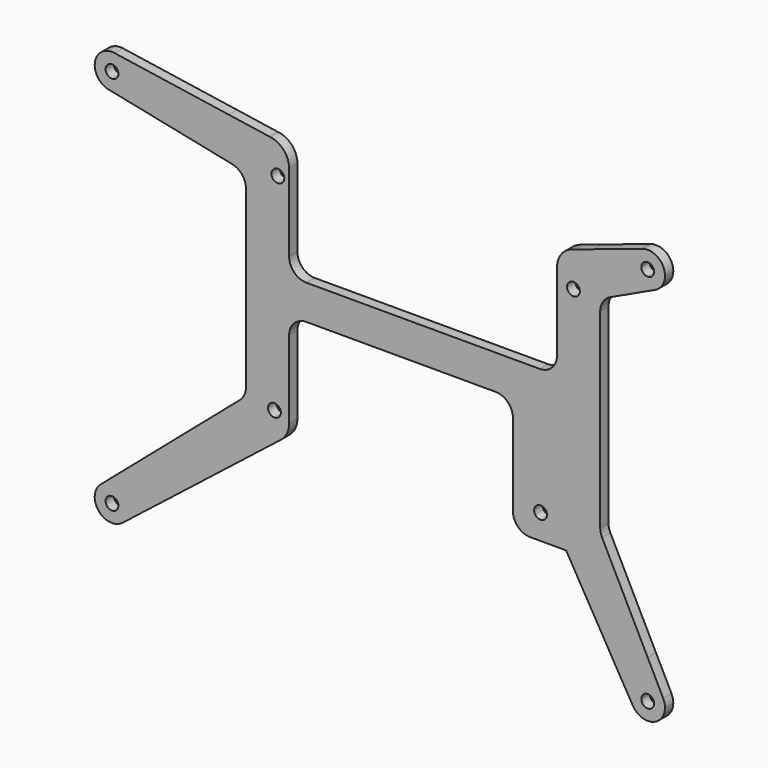
from build123d import *

# Parameters (mm, degrees)
F1_DEPTH = 3


# Not quite as in the source:
# - a feature names something its author has since deleted; it is built from what else it names


with BuildPart() as f1:
    # F0 (on Front) → F1 (new body)
    with BuildSketch(Plane.XZ):
        with BuildLine():
            Line((-37.214977254, 55.4332367199), (-65.9893809259, 55.4332367199))
            ThreePointArc((-65.9893809259, 55.4332367199), (-67.45384702, 51.8977028139), (-70.9893809259, 50.4332367199))
            Line((-70.9893809259, 50.4332367199), (-70.9893809259, 50.3281080825))
            Line((-70.9893809259, 50.3281080825), (-36.2299078147, 43.1628040761))
            ThreePointArc((-36.2299078147, 43.1628040761), (-33.3633413521, 41.4242986902), (-32.2393809259, 38.2657678257))
            Line((-32.2393809259, 38.2657678257), (-32.2393809259, -12.3991493743))
            ThreePointArc((-32.2393809259, -12.3991493743), (-32.6957967743, -14.4862150316), (-33.9817181489, -16.1922527517))
            Line((-33.9817181489, -16.1922527517), (-70.9893809259, -47.9758540661))
            Line((-70.9893809259, -47.9758540661), (-70.9893809259, -49.5667632801))
            ThreePointArc((-70.9893809259, -49.5667632801), (-67.45384702, -51.0312293742), (-65.9893809259, -54.5667632801))
            Line((-65.9893809259, -54.5667632801), (-62.9038139694, -54.5667632801))
            Line((-62.9038139694, -54.5667632801), (-22.1244695142, -22.4784798619))
            ThreePointArc((-22.1244695142, -22.4784798619), (-31.8953409933, -19.6117903415), (-25.9893809259, -11.3167632801))
            Line((-25.9893809259, -11.3167632801), (-25.9893809259, 41.1832367199))
            ThreePointArc((-25.9893809259, 41.1832367199), (-32.2393809259, 47.4332367199), (-25.9893809259, 53.6832367199))
            Line((-25.9893809259, 53.6832367199), (-25.5241895532, 53.6832367199))
            Line((-25.5241895532, 53.6832367199), (-37.214977254, 55.4332367199))
        make_face()
        with BuildLine():
            ThreePointArc((-70.2491754069, 60.3781427644), (-67.2011737249, 58.6965917729), (-65.9893809259, 55.4332367199))
            Line((-65.9893809259, 55.4332367199), (-37.214977254, 55.4332367199))
            Line((-37.214977254, 55.4332367199), (-70.2491754069, 60.3781427644))
        make_face()
        with BuildLine():
            ThreePointArc((-19.7393809259, 47.4332367199), (-21.2541219247, 51.5124305362), (-25.0641240271, 53.6143692756))
            ThreePointArc((-25.0641240271, 53.6143692756), (-25.5254727848, 53.6659960796), (-25.9893809259, 53.6832367199))
            ThreePointArc((-25.9893809259, 53.6832367199), (-32.2393809259, 47.4332367199), (-25.9893809259, 41.1832367199))
            ThreePointArc((-25.9893809259, 41.1832367199), (-21.5699635435, 43.0138193375), (-19.7393809259, 47.4332367199))
        make_face()
        with BuildLine():
            ThreePointArc((-21.1351809259, 44.4332367199), (-24.3004983196, 43.1221193262), (-22.9893809259, 46.2874367199))
            ThreePointArc((-22.9893809259, 46.2874367199), (-21.6782635322, 45.7443541135), (-21.1351809259, 44.4332367199))
        make_face(mode=Mode.SUBTRACT)
        with BuildLine():
            Line((-19.7393809259, 24.9332367629), (-19.7393809259, 47.4332367199))
            ThreePointArc((-19.7393809259, 47.4332367199), (-21.5699635435, 43.0138193375), (-25.9893809259, 41.1832367199))
            Line((-25.9893809259, 41.1832367199), (-25.9893809259, -11.3167632801))
            ThreePointArc((-25.9893809259, -11.3167632801), (-21.5699635435, -13.1473458977), (-19.7393809259, -17.5667632801))
            Line((-19.7393809259, -17.5667632801), (-19.7393809259, 4.9332367199))
            ThreePointArc((-19.7393809259, 4.9332367199), (-18.2749148318, 8.4687706258), (-14.7393809259, 9.9332367199))
            Line((-14.7393809259, 9.9332367199), (40.0127460063, 9.9332367199))
            ThreePointArc((40.0127460063, 9.9332367199), (43.5482799122, 8.4687706258), (45.0127460063, 4.9332367199))
            Line((45.0127460063, 4.9332367199), (45.0127460063, -17.5667632801))
            Line((45.0127460063, -17.5667632801), (51.449190997, -17.5667632801))
            ThreePointArc((51.449190997, -17.5667632801), (52.4896307348, -14.7872608805), (54.8648190741, -16.5667632801))
            ThreePointArc((54.8648190741, -16.5667632801), (54.7901214737, -17.0877516195), (54.5720471512, -17.5667632801))
            Line((54.5720471512, -17.5667632801), (57.7606190741, -17.5667632801))
            ThreePointArc((57.7606190741, -17.5667632801), (59.5912016917, -13.1473458977), (64.0106190741, -11.3167632801))
            Line((64.0106190741, -11.3167632801), (64.0106190741, 41.1832367199))
            ThreePointArc((64.0106190741, 41.1832367199), (59.5912016917, 43.0138193375), (57.7606190741, 47.4332367199))
            Line((57.7606190741, 47.4332367199), (57.7606190741, 24.9332367629))
            ThreePointArc((57.7606190741, 24.9332367629), (56.29615298, 21.3977028569), (52.7606190741, 19.9332367629))
            Line((52.7606190741, 19.9332367629), (-14.7393809259, 19.9332367629))
            ThreePointArc((-14.7393809259, 19.9332367629), (-18.2749148318, 21.3977028569), (-19.7393809259, 24.9332367629))
        make_face()
        with BuildLine():
            Line((-25.9893809259, -17.5667632801), (-25.9893809259, -11.3167632801))
            ThreePointArc((-25.9893809259, -11.3167632801), (-31.8953409933, -19.6117903415), (-22.1244695142, -22.4784798619))
            ThreePointArc((-22.1244695142, -22.4784798619), (-20.36718401, -20.2968551904), (-19.7393809259, -17.5667632801))
            Line((-19.7393809259, -17.5667632801), (-23.9893809259, -17.5667632801))
            Line((-23.9893809259, -17.5667632801), (-25.9893809259, -17.5667632801))
        make_face()
        with BuildLine():
            ThreePointArc((-19.7393809259, -17.5667632801), (-21.5699635435, -13.1473458977), (-25.9893809259, -11.3167632801))
            Line((-25.9893809259, -11.3167632801), (-25.9893809259, -17.5667632801))
            Line((-25.9893809259, -17.5667632801), (-23.9893809259, -17.5667632801))
            Line((-23.9893809259, -17.5667632801), (-19.7393809259, -17.5667632801))
        make_face()
        with BuildLine():
            ThreePointArc((-22.1351809259, -15.5667632801), (-22.6782635322, -16.8778806738), (-23.9893809259, -17.4209632801))
            ThreePointArc((-23.9893809259, -17.4209632801), (-25.3004983196, -14.2556458865), (-22.1351809259, -15.5667632801))
        make_face(mode=Mode.SUBTRACT)
        with BuildLine():
            Line((-62.9038139694, -54.5667632801), (-65.9893809259, -54.5667632801))
            ThreePointArc((-65.9893809259, -54.5667632801), (-66.4916233931, -56.7508368083), (-67.8974517965, -58.4961365456))
            Line((-67.8974517965, -58.4961365456), (-62.9038139694, -54.5667632801))
        make_face()
        with BuildLine():
            Line((-70.9893809259, -49.5667632801), (-70.9893809259, -47.9758540661))
            Line((-70.9893809259, -47.9758540661), (-74.2470437029, -50.7736599027))
            ThreePointArc((-74.2470437029, -50.7736599027), (-72.7264018114, -49.8781858367), (-70.9893809259, -49.5667632801))
        make_face()
        with BuildLine():
            Line((51.449190997, -17.5667632801), (45.0127460063, -17.5667632801))
            Line((45.0127460063, -17.5667632801), (45.0127460063, -18.8167632801))
            ThreePointArc((45.0127460063, -18.8167632801), (46.4772121003, -22.3522971861), (50.0127460063, -23.8167632801))
            Line((50.0127460063, -23.8167632801), (60.4091643842, -23.8167632801))
            Line((60.4091643842, -23.8167632801), (58.6032088142, -20.7008363936))
            ThreePointArc((58.6032088142, -20.7008363936), (57.974941228, -19.1894440675), (57.7606190741, -17.5667632801))
            Line((57.7606190741, -17.5667632801), (54.5720471512, -17.5667632801))
            ThreePointArc((54.5720471512, -17.5667632801), (53.0106190741, -18.4209632801), (51.449190997, -17.5667632801))
        make_face()
        with BuildLine():
            ThreePointArc((64.0106190741, 53.6832367199), (63.0073411856, 53.6021858588), (62.0300845889, 53.361135433))
            ThreePointArc((62.0300845889, 53.361135433), (58.9390887068, 51.0859178904), (57.7606190741, 47.4332367199))
            Line((57.7606190741, 47.4332367199), (64.0106190741, 47.4332367199))
            Line((64.0106190741, 47.4332367199), (70.2606190741, 47.4332367199))
            ThreePointArc((70.2606190741, 47.4332367199), (68.4300364565, 51.8526541023), (64.0106190741, 53.6832367199))
        make_face()
        with BuildLine():
            Line((82.4261914859, 60.1755556903), (68.2320500904, 55.4332367199))
            Line((68.2320500904, 55.4332367199), (79.0106190741, 55.4332367199))
            ThreePointArc((79.0106190741, 55.4332367199), (79.9533947803, 58.3553816563), (82.4261914859, 60.1755556903))
        make_face()
        with BuildLine():
            Line((79.0106190741, 55.4332367199), (68.2320500904, 55.4332367199))
            Line((68.2320500904, 55.4332367199), (62.9941595991, 53.6832367199))
            Line((62.9941595991, 53.6832367199), (64.0106190741, 53.6832367199))
            ThreePointArc((64.0106190741, 53.6832367199), (68.4300364565, 51.8526541023), (70.2606190741, 47.4332367199))
            Line((70.2606190741, 47.4332367199), (78.7288252988, 47.4332367199))
            Line((78.7288252988, 47.4332367199), (84.0106190741, 49.9105738121))
            Line((84.0106190741, 49.9105738121), (84.0106190741, 50.4332367199))
            ThreePointArc((84.0106190741, 50.4332367199), (80.4750851682, 51.8977028139), (79.0106190741, 55.4332367199))
        make_face()
        with BuildLine():
            Line((78.7288252988, 47.4332367199), (70.2606190741, 47.4332367199))
            ThreePointArc((70.2606190741, 47.4332367199), (68.4300364565, 43.0138193375), (64.0106190741, 41.1832367199))
            Line((64.0106190741, 41.1832367199), (64.0106190741, -11.3167632801))
            ThreePointArc((64.0106190741, -11.3167632801), (68.4300364565, -13.1473458977), (70.2606190741, -17.5667632801))
            ThreePointArc((70.2606190741, -17.5667632801), (68.4300364565, -21.9861806625), (64.0106190741, -23.8167632801))
            Line((64.0106190741, -23.8167632801), (60.4091643842, -23.8167632801))
            Line((60.4091643842, -23.8167632801), (78.2315125337, -54.5667632801))
            Line((78.2315125337, -54.5667632801), (79.0106190741, -54.5667632801))
            ThreePointArc((79.0106190741, -54.5667632801), (80.4750851682, -51.0312293742), (84.0106190741, -49.5667632801))
            Line((84.0106190741, -49.5667632801), (84.0106190741, -43.4349288765))
            Line((84.0106190741, -43.4349288765), (70.7933680849, -17.1438614305))
            ThreePointArc((70.7933680849, -17.1438614305), (70.3956290974, -16.0521179023), (70.2606190741, -14.898050085))
            Line((70.2606190741, -14.898050085), (70.2606190741, 40.2838696489))
            ThreePointArc((70.2606190741, 40.2838696489), (71.0406603386, 42.965650451), (73.1373983825, 44.810671378))
            Line((73.1373983825, 44.810671378), (78.7288252988, 47.4332367199))
        make_face()
        with BuildLine():
            Line((64.0106190741, 47.4332367199), (57.7606190741, 47.4332367199))
            ThreePointArc((57.7606190741, 47.4332367199), (59.5912016917, 43.0138193375), (64.0106190741, 41.1832367199))
            Line((64.0106190741, 41.1832367199), (64.0106190741, 42.3432561512))
            ThreePointArc((64.0106190741, 42.3432561512), (60.6564190741, 43.4332367199), (64.0106190741, 44.5232172885))
            Line((64.0106190741, 44.5232172885), (64.0106190741, 47.4332367199))
        make_face()
        with BuildLine():
            Line((64.0106190741, -17.5667632801), (64.0106190741, -11.3167632801))
            ThreePointArc((64.0106190741, -11.3167632801), (59.5912016917, -13.1473458977), (57.7606190741, -17.5667632801))
            Line((57.7606190741, -17.5667632801), (64.0106190741, -17.5667632801))
        make_face()
        with BuildLine():
            ThreePointArc((70.2606190741, -17.5667632801), (68.4300364565, -13.1473458977), (64.0106190741, -11.3167632801))
            Line((64.0106190741, -11.3167632801), (64.0106190741, -17.5667632801))
            Line((64.0106190741, -17.5667632801), (57.7606190741, -17.5667632801))
            ThreePointArc((57.7606190741, -17.5667632801), (57.974941228, -19.1894440675), (58.6032088142, -20.7008363936))
            ThreePointArc((58.6032088142, -20.7008363936), (60.8901589285, -22.9820406026), (64.0106190741, -23.8167632801))
            ThreePointArc((64.0106190741, -23.8167632801), (68.4300364565, -21.9861806625), (70.2606190741, -17.5667632801))
        make_face()
        with BuildLine():
            Line((58.6032088142, -20.7008363936), (60.4091643842, -23.8167632801))
            Line((60.4091643842, -23.8167632801), (64.0106190741, -23.8167632801))
            ThreePointArc((64.0106190741, -23.8167632801), (60.8901589285, -22.9820406026), (58.6032088142, -20.7008363936))
        make_face()
        with BuildLine():
            Line((88.4778700633, -52.3209519346), (84.0106190741, -43.4349288765))
            Line((84.0106190741, -43.4349288765), (84.0106190741, -49.5667632801))
            ThreePointArc((84.0106190741, -49.5667632801), (86.6346372974, -50.3106466976), (88.4778700633, -52.3209519346))
        make_face()
        with BuildLine():
            ThreePointArc((-70.9893809259, 53.5790367199), (-72.3004983196, 56.7443541135), (-69.1351809259, 55.4332367199))
            Line((-69.1351809259, 55.4332367199), (-65.9893809259, 55.4332367199))
            ThreePointArc((-65.9893809259, 55.4332367199), (-67.2011737249, 58.6965917729), (-70.2491754069, 60.3781427644))
            ThreePointArc((-70.2491754069, 60.3781427644), (-75.9121934648, 56.3084033935), (-71.9988540371, 50.5362004695))
            ThreePointArc((-71.9988540371, 50.5362004695), (-71.4967361998, 50.4590442602), (-70.9893809259, 50.4332367199))
            Line((-70.9893809259, 50.4332367199), (-70.9893809259, 53.5790367199))
        make_face()
        with BuildLine():
            Line((-65.9893809259, 55.4332367199), (-69.1351809259, 55.4332367199))
            ThreePointArc((-69.1351809259, 55.4332367199), (-69.6782635322, 54.1221193262), (-70.9893809259, 53.5790367199))
            Line((-70.9893809259, 53.5790367199), (-70.9893809259, 50.4332367199))
            ThreePointArc((-70.9893809259, 50.4332367199), (-67.45384702, 51.8977028139), (-65.9893809259, 55.4332367199))
        make_face()
        with BuildLine():
            ThreePointArc((82.4261914859, 60.1755556903), (79.9533947803, 58.3553816563), (79.0106190741, 55.4332367199))
            Line((79.0106190741, 55.4332367199), (82.1564190741, 55.4332367199))
            ThreePointArc((82.1564190741, 55.4332367199), (84.0106190741, 57.2874367199), (85.8648190741, 55.4332367199))
            ThreePointArc((85.8648190741, 55.4332367199), (85.3217364678, 54.1221193262), (84.0106190741, 53.5790367199))
            Line((84.0106190741, 53.5790367199), (84.0106190741, 50.4332367199))
            ThreePointArc((84.0106190741, 50.4332367199), (85.0982751214, 50.5529698908), (86.1338397657, 50.9064349908))
            ThreePointArc((86.1338397657, 50.9064349908), (88.2305778096, 52.7514559177), (89.0106190741, 55.4332367199))
            ThreePointArc((89.0106190741, 55.4332367199), (86.9327640105, 59.4904610137), (82.4261914859, 60.1755556903))
        make_face()
        with BuildLine():
            Line((82.1564190741, 55.4332367199), (79.0106190741, 55.4332367199))
            ThreePointArc((79.0106190741, 55.4332367199), (80.4750851682, 51.8977028139), (84.0106190741, 50.4332367199))
            Line((84.0106190741, 50.4332367199), (84.0106190741, 53.5790367199))
            ThreePointArc((84.0106190741, 53.5790367199), (82.6995016804, 54.1221193262), (82.1564190741, 55.4332367199))
        make_face()
        with BuildLine():
            ThreePointArc((-65.9893809259, -54.5667632801), (-67.45384702, -51.0312293742), (-70.9893809259, -49.5667632801))
            Line((-70.9893809259, -49.5667632801), (-70.9893809259, -52.7125632801))
            ThreePointArc((-70.9893809259, -52.7125632801), (-69.6782635322, -53.2556458865), (-69.1351809259, -54.5667632801))
            Line((-69.1351809259, -54.5667632801), (-65.9893809259, -54.5667632801))
        make_face()
        with BuildLine():
            Line((-70.9893809259, -52.7125632801), (-70.9893809259, -49.5667632801))
            ThreePointArc((-70.9893809259, -49.5667632801), (-72.7264018114, -49.8781858367), (-74.2470437029, -50.7736599027))
            ThreePointArc((-74.2470437029, -50.7736599027), (-74.8515083558, -57.7422902781), (-67.8974517965, -58.4961365456))
            ThreePointArc((-67.8974517965, -58.4961365456), (-66.4916233931, -56.7508368083), (-65.9893809259, -54.5667632801))
            Line((-65.9893809259, -54.5667632801), (-69.1351809259, -54.5667632801))
            ThreePointArc((-69.1351809259, -54.5667632801), (-72.3004983196, -55.8778806738), (-70.9893809259, -52.7125632801))
        make_face()
        with BuildLine():
            ThreePointArc((84.0106190741, -49.5667632801), (80.4750851682, -51.0312293742), (79.0106190741, -54.5667632801))
            Line((79.0106190741, -54.5667632801), (82.1564190741, -54.5667632801))
            ThreePointArc((82.1564190741, -54.5667632801), (82.6995016804, -53.2556458865), (84.0106190741, -52.7125632801))
            Line((84.0106190741, -52.7125632801), (84.0106190741, -49.5667632801))
        make_face()
        with BuildLine():
            Line((82.1564190741, -54.5667632801), (79.0106190741, -54.5667632801))
            ThreePointArc((79.0106190741, -54.5667632801), (79.1820767972, -55.86490791), (79.6846908662, -57.0740217709))
            ThreePointArc((79.6846908662, -57.0740217709), (85.308763704, -59.395305557), (89.0106190741, -54.5667632801))
            ThreePointArc((89.0106190741, -54.5667632801), (88.8756090508, -53.4126954628), (88.4778700633, -52.3209519346))
            ThreePointArc((88.4778700633, -52.3209519346), (86.6346372974, -50.3106466976), (84.0106190741, -49.5667632801))
            Line((84.0106190741, -49.5667632801), (84.0106190741, -52.7125632801))
            ThreePointArc((84.0106190741, -52.7125632801), (85.3217364678, -53.2556458865), (85.8648190741, -54.5667632801))
            ThreePointArc((85.8648190741, -54.5667632801), (84.0106190741, -56.4209632801), (82.1564190741, -54.5667632801))
        make_face()
        with BuildLine():
            Line((79.0106190741, -54.5667632801), (78.2315125337, -54.5667632801))
            Line((78.2315125337, -54.5667632801), (79.6846908662, -57.0740217709))
            ThreePointArc((79.6846908662, -57.0740217709), (79.1820767972, -55.86490791), (79.0106190741, -54.5667632801))
        make_face()
        with BuildLine():
            ThreePointArc((86.1338397657, 50.9064349908), (85.0982751214, 50.5529698908), (84.0106190741, 50.4332367199))
            Line((84.0106190741, 50.4332367199), (84.0106190741, 49.9105738121))
            Line((84.0106190741, 49.9105738121), (86.1338397657, 50.9064349908))
        make_face()
        with BuildLine():
            Line((64.0106190741, 53.6832367199), (62.9941595991, 53.6832367199))
            Line((62.9941595991, 53.6832367199), (62.0300845889, 53.361135433))
            ThreePointArc((62.0300845889, 53.361135433), (63.0073411856, 53.6021858588), (64.0106190741, 53.6832367199))
        make_face()
        with BuildLine():
            Line((-70.9893809259, 50.3281080825), (-70.9893809259, 50.4332367199))
            ThreePointArc((-70.9893809259, 50.4332367199), (-71.4967361998, 50.4590442602), (-71.9988540371, 50.5362004695))
            Line((-71.9988540371, 50.5362004695), (-70.9893809259, 50.3281080825))
        make_face()
        with BuildLine():
            Line((-25.0641240271, 53.6143692756), (-25.5241895532, 53.6832367199))
            Line((-25.5241895532, 53.6832367199), (-25.9893809259, 53.6832367199))
            ThreePointArc((-25.9893809259, 53.6832367199), (-25.5254727848, 53.6659960796), (-25.0641240271, 53.6143692756))
        make_face()
        with BuildLine():
            ThreePointArc((64.0106190741, 41.1832367199), (68.4300364565, 43.0138193375), (70.2606190741, 47.4332367199))
            Line((70.2606190741, 47.4332367199), (64.0106190741, 47.4332367199))
            Line((64.0106190741, 47.4332367199), (64.0106190741, 44.5232172885))
            ThreePointArc((64.0106190741, 44.5232172885), (64.2740472184, 44.0062801912), (64.3648190741, 43.4332367199))
            ThreePointArc((64.3648190741, 43.4332367199), (64.2740472184, 42.8601932486), (64.0106190741, 42.3432561512))
            Line((64.0106190741, 42.3432561512), (64.0106190741, 41.1832367199))
        make_face()
    extrude(amount=F1_DEPTH)


solid = f1.part
